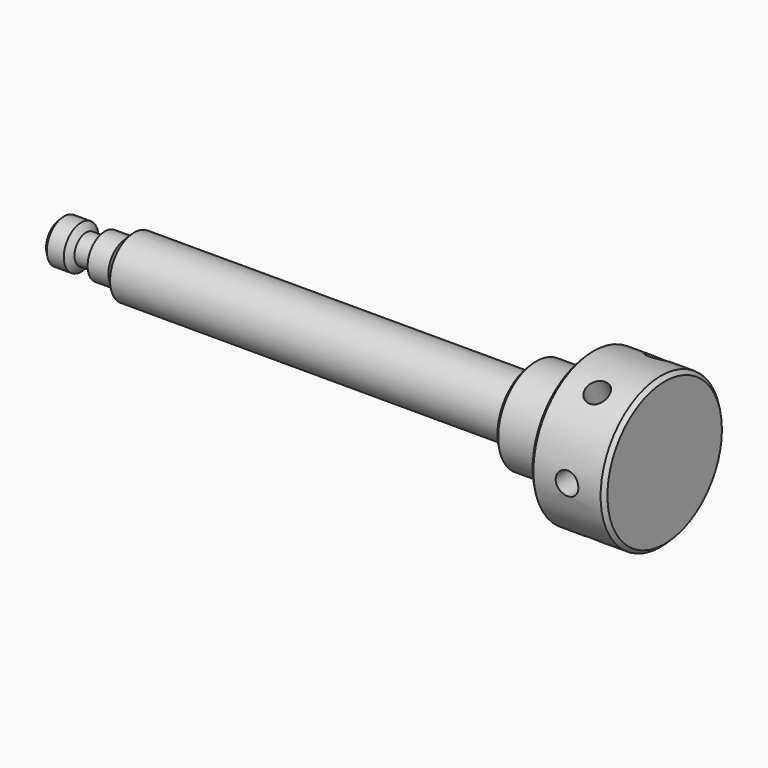
from build123d import *

# Parameters (mm, degrees)
F2_SIZE   = 1
F3_SIZE   = 2.24999
F17_D     = 6
F17_DEPTH = 8
F17_TIP   = 1.8025818571
F18_D     = 6
F18_DEPTH = 8
F18_TIP   = 1.8025818571
F19_D     = 6
F19_DEPTH = 8
F19_TIP   = 1.8025818571
F20_D     = 6
F20_DEPTH = 8
F20_TIP   = 1.8025818571
F21_D     = 6
F21_DEPTH = 8
F21_TIP   = 1.8025818571
F22_D     = 6
F22_DEPTH = 8
F22_TIP   = 1.8025818571


# Not quite as in the source:
# - a fillet or chamfer is up to 0.001 mm smaller than in the source, because OpenCascade refuses the exact size


with BuildPart() as f1:
    # F0 (on Top) → F1 (revolve)
    with BuildSketch(Plane.XY):
        Polygon((-160, 0), (0, 0), (0, 19.95), (-19.8, 19.95), (-19.8, 12.6), (-35, 12.6), (-35, 8), (-142.7, 8), (-142.7, 5.75), (-148.2, 5.75), (-148.2, 3.85), (-153.2, 3.85), (-154.5, 5.75), (-160, 5.75), align=None)
    revolve(axis=Axis((-80, 0, 0), (1, 0, 0)))

    # F2
    f2_edges = [f1.edges().sort_by_distance(p)[0] for p in [
        (-160, -5.75, 0),
        (0, -19.95, 0),
        (-35, -12.6, 0),
        (-19.8, -19.95, 0),
    ]]
    chamfer(f2_edges, length=F2_SIZE)

    # F3 (size 2.25 in the source; OpenCascade refuses exactly that, so slightly less here)
    f3_edges = [f1.edges().sort_by_distance(p)[0] for p in [
        (-142.7, -8, 0),
    ]]
    chamfer(f3_edges, length=F3_SIZE)

    # F17
    with Locations(Plane(origin=(0, -19.95, 0), x_dir=(-1, 0, 0), z_dir=(0, -1, 0))):
        with Locations((9.9, 0)):
            Hole(F17_D / 2, depth=F17_DEPTH)
            with Locations((0, 0, -(F17_DEPTH + F17_TIP / 2))):  # 118° drill point
                Cone(0, F17_D / 2, F17_TIP, mode=Mode.SUBTRACT)

    # F18
    with Locations(Plane(origin=(0, -9.975, 17.2772068055), x_dir=(1, 0, 0), z_dir=(0, -0.5, 0.8660254038))):
        with Locations((-9.9, 0)):
            Hole(F18_D / 2, depth=F18_DEPTH)
            with Locations((0, 0, -(F18_DEPTH + F18_TIP / 2))):  # 118° drill point
                Cone(0, F18_D / 2, F18_TIP, mode=Mode.SUBTRACT)

    # F19
    with Locations(Plane(origin=(0, 9.975, 17.2772068055), x_dir=(1, 0, 0), z_dir=(0, 0.5, 0.8660254038))):
        with Locations((-9.9, 0)):
            Hole(F19_D / 2, depth=F19_DEPTH)
            with Locations((0, 0, -(F19_DEPTH + F19_TIP / 2))):  # 118° drill point
                Cone(0, F19_D / 2, F19_TIP, mode=Mode.SUBTRACT)

    # F20
    with Locations(Plane(origin=(0, 19.95, 0), x_dir=(-1, 0, 0), z_dir=(0, 1, 0))):
        with Locations((9.9, 0)):
            Hole(F20_D / 2, depth=F20_DEPTH)
            with Locations((0, 0, -(F20_DEPTH + F20_TIP / 2))):  # 118° drill point
                Cone(0, F20_D / 2, F20_TIP, mode=Mode.SUBTRACT)

    # F21
    with Locations(Plane(origin=(0, 9.975, -17.2772068055), x_dir=(1, 0, 0), z_dir=(0, 0.5, -0.8660254038))):
        with Locations((-9.9, 0)):
            Hole(F21_D / 2, depth=F21_DEPTH)
            with Locations((0, 0, -(F21_DEPTH + F21_TIP / 2))):  # 118° drill point
                Cone(0, F21_D / 2, F21_TIP, mode=Mode.SUBTRACT)

    # F22
    with Locations(Plane(origin=(0, -9.975, -17.2772068055), x_dir=(1, 0, 0), z_dir=(0, -0.5, -0.8660254038))):
        with Locations((-9.9, 0)):
            Hole(F22_D / 2, depth=F22_DEPTH)
            with Locations((0, 0, -(F22_DEPTH + F22_TIP / 2))):  # 118° drill point
                Cone(0, F22_D / 2, F22_TIP, mode=Mode.SUBTRACT)


solid = f1.part
